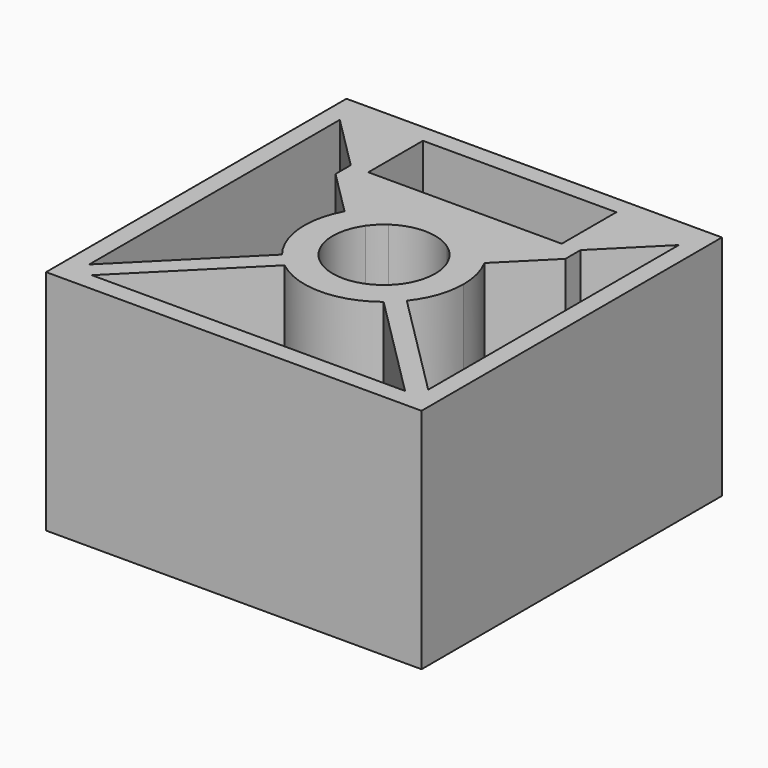
from build123d import *

# Parameters (mm, degrees)
F0_W     = 16.5
F0_H     = 16.5
F1_DEPTH = 10


# Not quite as in the source:
# - a feature names something its author has since deleted; it is built from what else it names


with BuildPart() as f1:
    # F0 (on Top) → F1 (new body)
    with BuildSketch(Plane.XY):
        Rectangle(F0_W, F0_H)
        Polygon((6.8843145751, 7.45), (7.45, 7.45), (7.45, 6.8843145751), (7.45, -6.8843145751), (7.45, -7.45), (6.8843145751, -7.45), (-6.8843145751, -7.45), (-7.45, -7.45), (-7.45, -6.8843145751), (-7.45, 6.8843145751), (-7.45, 7.45), (-6.8843145751, 7.45), (-5.05, 7.45), (-4.25, 7.45), (4.25, 7.45), (5.05, 7.45), align=None, mode=Mode.SUBTRACT)
        Polygon((-4.25, 4.8156854249), (-4.25, 7.45), (-5.05, 7.45), (-5.05, 5.6156854249), align=None)
        Polygon((-4.25, 4.45), (-4.25, 4.8156854249), (-5.05, 5.6156854249), (-5.05, 4.4843145751), (-4.2156854249, 3.65), (-3.0843145751, 3.65), (-3.8843145751, 4.45), align=None)
        Polygon((7.45, 6.8843145751), (7.45, 7.45), (6.8843145751, 7.45), (5.05, 5.6156854249), (5.05, 4.4843145751), align=None)
        Polygon((-5.05, 5.6156854249), (-6.8843145751, 7.45), (-7.45, 7.45), (-7.45, 6.8843145751), (-5.05, 4.4843145751), align=None)
        with BuildLine():
            Line((-1.2828041187, 1.8484895437), (-2.1758154582, 2.7415008831))
            ThreePointArc((-2.1758154582, 2.7415008831), (-2.4748737342, 2.4748737342), (-2.7415008831, 2.1758154582))
            Line((-2.7415008831, 2.1758154582), (-1.8484895437, 1.2828041187))
            ThreePointArc((-1.8484895437, 1.2828041187), (-1.5909902577, 1.5909902577), (-1.2828041187, 1.8484895437))
        make_face()
        with BuildLine():
            ThreePointArc((-3.0738154941, 1.6738154941), (-3.4870317978, -0.3010136893), (-2.7415008831, -2.1758154582))
            Line((-2.7415008831, -2.1758154582), (-1.8484895437, -1.2828041187))
            ThreePointArc((-1.8484895437, -1.2828041187), (-2.25, 0), (-1.8484895437, 1.2828041187))
            Line((-1.8484895437, 1.2828041187), (-2.7415008831, 2.1758154582))
            ThreePointArc((-2.7415008831, 2.1758154582), (-2.9184717118, 1.9319738268), (-3.0738154941, 1.6738154941))
        make_face()
        with BuildLine():
            ThreePointArc((-2.7415008831, -2.1758154582), (-2.4748737342, -2.4748737342), (-2.1758154582, -2.7415008831))
            Line((-2.1758154582, -2.7415008831), (-1.2828041187, -1.8484895437))
            ThreePointArc((-1.2828041187, -1.8484895437), (-1.5909902577, -1.5909902577), (-1.8484895437, -1.2828041187))
            Line((-1.8484895437, -1.2828041187), (-2.7415008831, -2.1758154582))
        make_face()
        with BuildLine():
            Line((-7.45, -7.45), (-6.8843145751, -7.45))
            Line((-6.8843145751, -7.45), (-2.1758154582, -2.7415008831))
            ThreePointArc((-2.1758154582, -2.7415008831), (-2.4748737342, -2.4748737342), (-2.7415008831, -2.1758154582))
            Line((-2.7415008831, -2.1758154582), (-7.45, -6.8843145751))
            Line((-7.45, -6.8843145751), (-7.45, -7.45))
        make_face()
        with BuildLine():
            ThreePointArc((-2.1758154582, -2.7415008831), (0, -3.5), (2.1758154582, -2.7415008831))
            Line((2.1758154582, -2.7415008831), (1.2828041187, -1.8484895437))
            ThreePointArc((1.2828041187, -1.8484895437), (0, -2.25), (-1.2828041187, -1.8484895437))
            Line((-1.2828041187, -1.8484895437), (-2.1758154582, -2.7415008831))
        make_face()
        with BuildLine():
            ThreePointArc((2.1758154582, -2.7415008831), (2.4748737342, -2.4748737342), (2.7415008831, -2.1758154582))
            Line((2.7415008831, -2.1758154582), (1.8484895437, -1.2828041187))
            ThreePointArc((1.8484895437, -1.2828041187), (1.5909902577, -1.5909902577), (1.2828041187, -1.8484895437))
            Line((1.2828041187, -1.8484895437), (2.1758154582, -2.7415008831))
        make_face()
        with BuildLine():
            Line((1.8484895437, -1.2828041187), (2.7415008831, -2.1758154582))
            ThreePointArc((2.7415008831, -2.1758154582), (3.3049397189, -1.1521169448), (3.5, 0))
            ThreePointArc((3.5, 0), (3.3917808176, 0.8636103782), (3.0738154941, 1.6738154941))
            ThreePointArc((3.0738154941, 1.6738154941), (2.9184717118, 1.9319738268), (2.7415008831, 2.1758154582))
            Line((2.7415008831, 2.1758154582), (1.8484895437, 1.2828041187))
            ThreePointArc((1.8484895437, 1.2828041187), (2.1472775174, 0.672085756), (2.25, 0))
            ThreePointArc((2.25, 0), (2.1472775174, -0.672085756), (1.8484895437, -1.2828041187))
        make_face()
        with BuildLine():
            Line((7.45, -7.45), (7.45, -6.8843145751))
            Line((7.45, -6.8843145751), (2.7415008831, -2.1758154582))
            ThreePointArc((2.7415008831, -2.1758154582), (2.4748737342, -2.4748737342), (2.1758154582, -2.7415008831))
            Line((2.1758154582, -2.7415008831), (6.8843145751, -7.45))
            Line((6.8843145751, -7.45), (7.45, -7.45))
        make_face()
        with BuildLine():
            Line((1.8484895437, 1.2828041187), (2.7415008831, 2.1758154582))
            ThreePointArc((2.7415008831, 2.1758154582), (2.4748737342, 2.4748737342), (2.1758154582, 2.7415008831))
            Line((2.1758154582, 2.7415008831), (1.2828041187, 1.8484895437))
            ThreePointArc((1.2828041187, 1.8484895437), (1.5909902577, 1.5909902577), (1.8484895437, 1.2828041187))
        make_face()
        Polygon((5.05, 4.4843145751), (5.05, 5.6156854249), (4.25, 4.8156854249), (4.25, 4.45), (3.8843145751, 4.45), (3.0843145751, 3.65), (4.2156854249, 3.65), align=None)
        Polygon((5.05, 3.65), (5.05, 4.4843145751), (4.2156854249, 3.65), align=None)
        Polygon((5.05, 5.6156854249), (5.05, 7.45), (4.25, 7.45), (4.25, 4.8156854249), align=None)
        Polygon((3.0843145751, 3.65), (3.8843145751, 4.45), (-3.8843145751, 4.45), (-3.0843145751, 3.65), align=None)
        Polygon((5.05, 5.6156854249), (6.8843145751, 7.45), (5.05, 7.45), align=None)
        Polygon((-5.05, 5.6156854249), (-5.05, 7.45), (-6.8843145751, 7.45), align=None)
        Polygon((-5.05, 3.65), (-4.2156854249, 3.65), (-5.05, 4.4843145751), align=None)
        with BuildLine():
            Line((2.1758154582, 2.7415008831), (3.0843145751, 3.65))
            Line((3.0843145751, 3.65), (-3.0843145751, 3.65))
            Line((-3.0843145751, 3.65), (-2.1758154582, 2.7415008831))
            ThreePointArc((-2.1758154582, 2.7415008831), (0, 3.5), (2.1758154582, 2.7415008831))
        make_face()
        with BuildLine():
            Line((-2.1758154582, 2.7415008831), (-3.0843145751, 3.65))
            Line((-3.0843145751, 3.65), (-4.2156854249, 3.65))
            Line((-4.2156854249, 3.65), (-2.7415008831, 2.1758154582))
            ThreePointArc((-2.7415008831, 2.1758154582), (-2.4748737342, 2.4748737342), (-2.1758154582, 2.7415008831))
        make_face()
        with BuildLine():
            Line((2.7415008831, 2.1758154582), (4.2156854249, 3.65))
            Line((4.2156854249, 3.65), (3.0843145751, 3.65))
            Line((3.0843145751, 3.65), (2.1758154582, 2.7415008831))
            ThreePointArc((2.1758154582, 2.7415008831), (2.4748737342, 2.4748737342), (2.7415008831, 2.1758154582))
        make_face()
        with BuildLine():
            Line((-2.7415008831, 2.1758154582), (-4.2156854249, 3.65))
            Line((-4.2156854249, 3.65), (-5.05, 3.65))
            Line((-5.05, 3.65), (-3.0738154941, 1.6738154941))
            ThreePointArc((-3.0738154941, 1.6738154941), (-2.9184717118, 1.9319738268), (-2.7415008831, 2.1758154582))
        make_face()
        with BuildLine():
            Line((3.0738154941, 1.6738154941), (5.05, 3.65))
            Line((5.05, 3.65), (4.2156854249, 3.65))
            Line((4.2156854249, 3.65), (2.7415008831, 2.1758154582))
            ThreePointArc((2.7415008831, 2.1758154582), (2.9184717118, 1.9319738268), (3.0738154941, 1.6738154941))
        make_face()
        with BuildLine():
            Line((1.2828041187, 1.8484895437), (2.1758154582, 2.7415008831))
            ThreePointArc((2.1758154582, 2.7415008831), (0, 3.5), (-2.1758154582, 2.7415008831))
            Line((-2.1758154582, 2.7415008831), (-1.2828041187, 1.8484895437))
            ThreePointArc((-1.2828041187, 1.8484895437), (0, 2.25), (1.2828041187, 1.8484895437))
        make_face()
    extrude(amount=F1_DEPTH)


solid = f1.part
